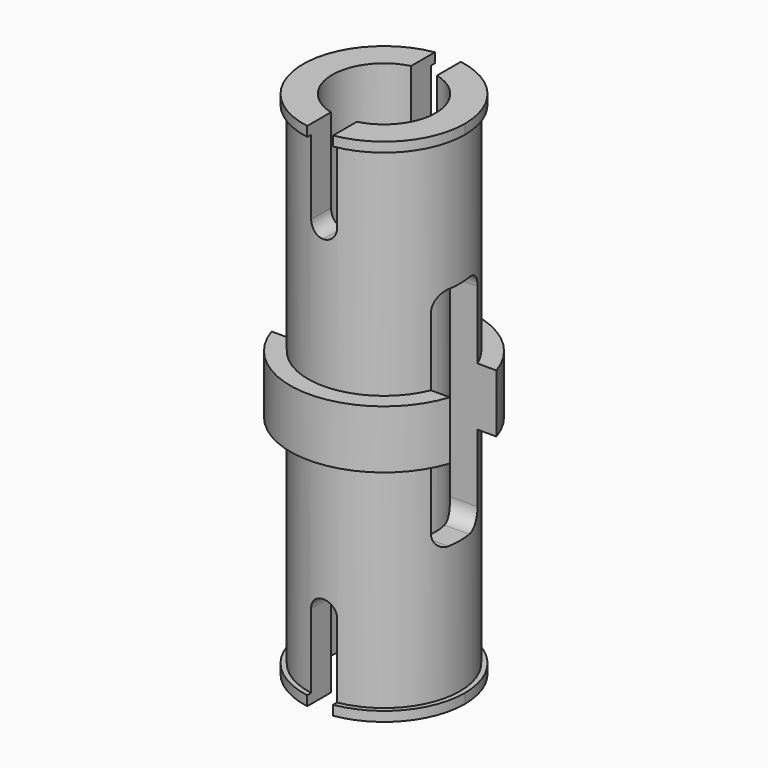
from build123d import *

# Parameters (mm, degrees)
F0_R      = 2.35
F0_R_2    = 1.6
F1_DEPTH  = 7.9
F3_DEPTH  = 3
F0_R_3    = 2.9
F4_DEPTH  = 0.9
F5_W      = 1.8
F5_H      = 7
F6_DEPTH  = 12.5
F7_R      = 0.5
F9_DEPTH  = 3
F10_R     = 0.3999
F12_DEPTH = 0.3
F14_DEPTH = 0.3
F16_DEPTH = 0.3


# Not quite as in the source:
# - a fillet or chamfer is up to 0.001 mm smaller than in the source, because OpenCascade refuses the exact size


with BuildPart() as f1:
    # F0 (on Top) → F1 (new body, symmetric)
    with BuildSketch(Plane.XY):
        Circle(F0_R)
        Circle(F0_R_2, mode=Mode.SUBTRACT)
    extrude(amount=F1_DEPTH, both=True)

    # F2 (on face) → F3 (cut)
    with BuildSketch(Plane.XY.offset(7.9)):
        with BuildLine():
            ThreePointArc((-0.4, 1.5491933385), (-0.201606868, 1.587247514), (0, 1.6))
            ThreePointArc((0, 1.6), (0.201606868, 1.587247514), (0.4, 1.5491933385))
            Line((0.4, 1.5491933385), (0.4, 1.6))
            Line((0.4, 1.6), (0.4, 2.3157072354))
            ThreePointArc((0.4, 2.3157072354), (0, 2.35), (-0.4, 2.3157072354))
            Line((-0.4, 2.3157072354), (-0.4, 1.6))
            Line((-0.4, 1.6), (-0.4, 1.5491933385))
        make_face()
        with BuildLine():
            ThreePointArc((0.4, -1.5491933385), (0.201606868, -1.587247514), (0, -1.6))
            ThreePointArc((0, -1.6), (-0.201606868, -1.587247514), (-0.4, -1.5491933385))
            Line((-0.4, -1.5491933385), (-0.4, -1.6))
            Line((-0.4, -1.6), (-0.4, -2.3157072354))
            ThreePointArc((-0.4, -2.3157072354), (0, -2.35), (0.4, -2.3157072354))
            Line((0.4, -2.3157072354), (0.4, -1.6))
            Line((0.4, -1.6), (0.4, -1.5491933385))
        make_face()
    extrude(amount=-F3_DEPTH, mode=Mode.SUBTRACT)

    # F0 (on Top) → F4 (join, symmetric)
    with BuildSketch(Plane.XY):
        Circle(F0_R_3)
        Circle(F0_R, mode=Mode.SUBTRACT)
    extrude(amount=F4_DEPTH, both=True)

    # F5 (on Right) → F6 (cut, symmetric)
    with BuildSketch(Plane.YZ):
        Rectangle(F5_W, F5_H)
    extrude(amount=F6_DEPTH, both=True, mode=Mode.SUBTRACT)

    # F7
    f7_edges = [f1.edges().sort_by_distance(p)[0] for p in [
        (-1.746852, -0.9, 3.5),
        (1.746852, -0.9, 3.5),
        (1.746852, 0.9, 3.5),
        (-1.746852, 0.9, 3.5),
        (1.746852, -0.9, -3.5),
        (-1.746852, -0.9, -3.5),
        (1.746852, 0.9, -3.5),
        (-1.746852, 0.9, -3.5),
    ]]
    fillet(f7_edges, radius=F7_R)

    # F8 (on face) → F9 (cut)
    with BuildSketch(Plane(origin=(0, 0, -7.9), x_dir=(1, 0, 0), z_dir=(0, 0, -1))):
        with BuildLine():
            Line((0.4, 1.5491933385), (0.4, 1.6))
            Line((0.4, 1.6), (0.4, 2.3157072354))
            ThreePointArc((0.4, 2.3157072354), (0, 2.35), (-0.4, 2.3157072354))
            Line((-0.4, 2.3157072354), (-0.4, 1.6))
            Line((-0.4, 1.6), (-0.4, 1.5491933385))
            ThreePointArc((-0.4, 1.5491933385), (0, 1.6), (0.4, 1.5491933385))
        make_face()
        with BuildLine():
            ThreePointArc((-0.4, -2.3157072354), (0, -2.35), (0.4, -2.3157072354))
            Line((0.4, -2.3157072354), (0.4, -1.6))
            Line((0.4, -1.6), (0.4, -1.5491933385))
            ThreePointArc((0.4, -1.5491933385), (0, -1.6), (-0.4, -1.5491933385))
            Line((-0.4, -1.5491933385), (-0.4, -1.6))
            Line((-0.4, -1.6), (-0.4, -2.3157072354))
        make_face()
    extrude(amount=-F9_DEPTH, mode=Mode.SUBTRACT)

    # F10 (radius 0.4 in the source; OpenCascade refuses exactly that, so slightly less here)
    f10_edges = [f1.edges().sort_by_distance(p)[0] for p in [
        (0.4, -1.93245, -4.9),
        (-0.4, -1.93245, -4.9),
        (-0.4, 1.93245, -4.9),
        (0.4, 1.93245, -4.9),
        (0.4, 1.93245, 4.9),
        (-0.4, 1.93245, 4.9),
        (-0.4, -1.93245, 4.9),
        (0.4, -1.93245, 4.9),
    ]]
    fillet(f10_edges, radius=F10_R)

    # F11 (on face) → F12 (join)
    with BuildSketch(Plane(origin=(0, 0, -7.9), x_dir=(1, 0, 0), z_dir=(0, 0, -1))):
        with BuildLine():
            Line((-0.4, 2.3157072354), (-0.4, 2.4677925359))
            ThreePointArc((-0.4, 2.4677925359), (-2.5, 0), (-0.4, -2.4677925359))
            Line((-0.4, -2.4677925359), (-0.4, -2.3157072354))
            ThreePointArc((-0.4, -2.3157072354), (-2.35, 0), (-0.4, 2.3157072354))
        make_face()
        with BuildLine():
            ThreePointArc((0.4, -2.4677925359), (1.9039432765, -1.6201851746), (2.5, 0))
            ThreePointArc((2.5, 0), (1.9039432765, 1.6201851746), (0.4, 2.4677925359))
            Line((0.4, 2.4677925359), (0.4, 2.3157072354))
            ThreePointArc((0.4, 2.3157072354), (1.7975678012, 1.5136875503), (2.35, 0))
            ThreePointArc((2.35, 0), (1.7975678012, -1.5136875503), (0.4, -2.3157072354))
            Line((0.4, -2.3157072354), (0.4, -2.4677925359))
        make_face()
    extrude(amount=-F12_DEPTH)

    # F13 (on face) → F14 (join)
    with BuildSketch(Plane.XY.offset(7.9)):
        with BuildLine():
            Line((-0.4, 2.3157072354), (-0.4, 2.4677925359))
            ThreePointArc((-0.4, 2.4677925359), (-2.5, 0), (-0.4, -2.4677925359))
            Line((-0.4, -2.4677925359), (-0.4, -2.3157072354))
            ThreePointArc((-0.4, -2.3157072354), (-2.35, 0), (-0.4, 2.3157072354))
        make_face()
    extrude(amount=-F14_DEPTH)

    # F15 (on face) → F16 (join)
    with BuildSketch(Plane.XY.offset(7.9)):
        with BuildLine():
            ThreePointArc((0.4, -2.4677925359), (1.9039432765, -1.6201851746), (2.5, 0))
            ThreePointArc((2.5, 0), (1.9039432765, 1.6201851746), (0.4, 2.4677925359))
            Line((0.4, 2.4677925359), (0.4, 2.3157072354))
            ThreePointArc((0.4, 2.3157072354), (1.7975678012, 1.5136875503), (2.35, 0))
            ThreePointArc((2.35, 0), (1.7975678012, -1.5136875503), (0.4, -2.3157072354))
            Line((0.4, -2.3157072354), (0.4, -2.4677925359))
        make_face()
    extrude(amount=-F16_DEPTH)


solid = f1.part
